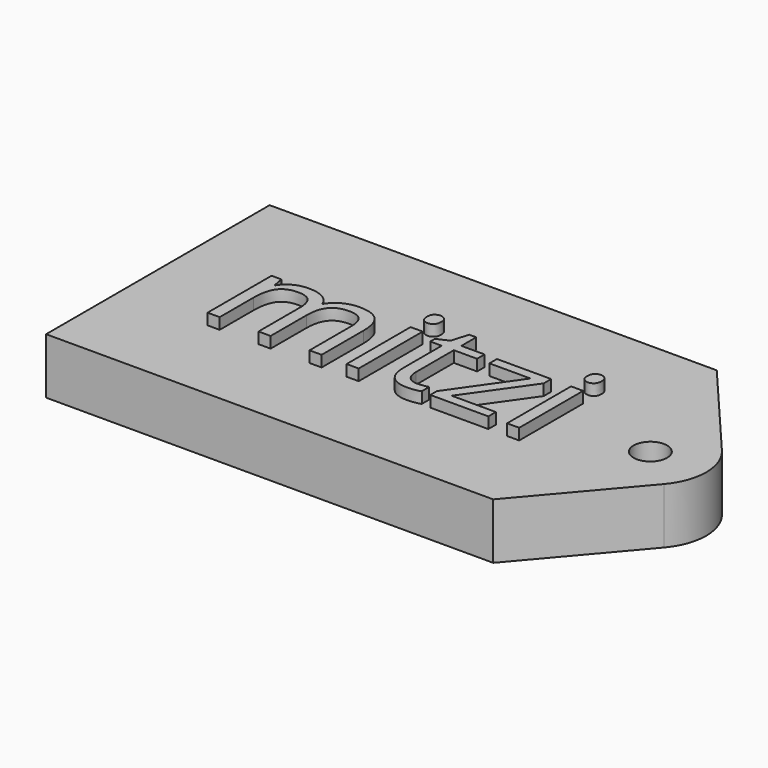
from build123d import *

# Parameters (mm, degrees)
F1_DEPTH     = 5
F2_R         = 5
F4_D         = 3
F5_TEXT_SIZE = 13.3714046939
F6_DEPTH     = 1


# Not quite as in the source:
# - Text() gives the source's letters only with a copy of the font that has no kerning and outlines rounded to 1/6400 em; it was checked with that copy


with BuildPart() as f1:
    # F0 (on Top) → F1 (new body)
    with BuildSketch(Plane.XY):
        Polygon((-20, -12.5), (20, -12.5), (30.6250024587, 0), (20, 12.5), (-20, 12.5), align=None)
    extrude(amount=F1_DEPTH)

    # F2
    f2_edges = [f1.edges().sort_by_distance(p)[0] for p in [
        (30.625002, 0, 2.5),
    ]]
    fillet(f2_edges, radius=F2_R)

    # F4 (through all)
    with Locations(Plane.XY.offset(5)):
        with Locations((24.0627994475, 0)):
            Hole(F4_D / 2)

    # F5 (on face) → F6 (join)
    with BuildSketch(Plane.XY.offset(5)):
        with Locations((-13.174759096, -4.409247674)):
            Text('mitzi', F5_TEXT_SIZE, font='Open Sans', text_align=(TextAlign.LEFT, TextAlign.BOTTOM))
    extrude(amount=F6_DEPTH)


solid = f1.part
